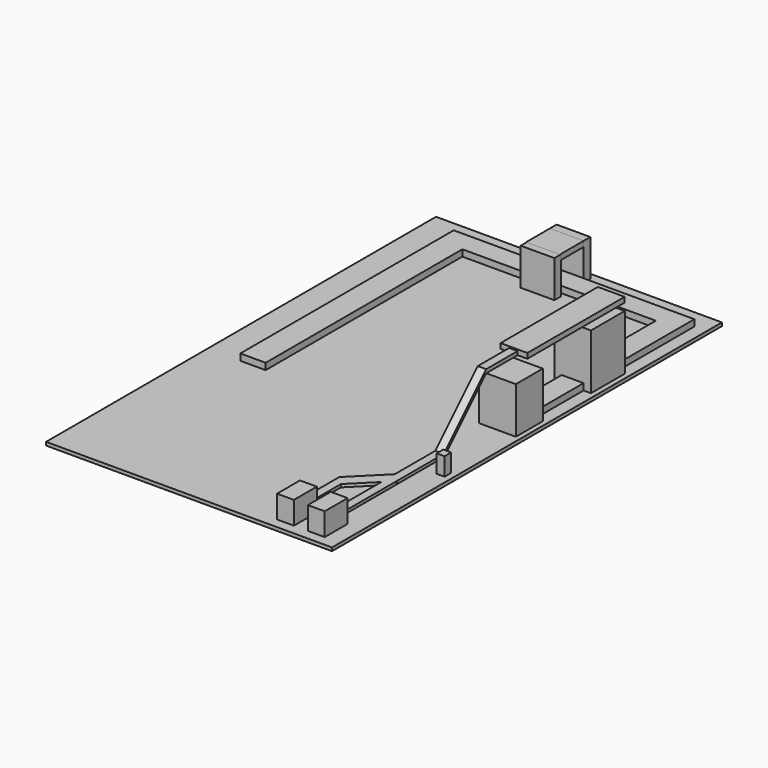
from build123d import *

# Parameters (mm, degrees)
F0_W         = 25.4
F0_H         = 43.18
F1_DEPTH     = 34.29
F4_DEPTH     = 186.69
F5_DEPTH     = 66.04
F6_SIZE      = 12.69999
F7_DEPTH     = 66.802
F8_W         = 11.9172371924
F8_H         = 12.5130861998
F9_DEPTH     = 27.178
F10_DEPTH    = 7.62
F11_T1_DEPTH = 38.8282991577
F12_W        = 12.7
F12_H        = 3.8690640952
F13_DEPTH    = 114.3
F14_T1_DEPTH = 38.8282991577
F15_DEPTH    = 59.182
F16_W        = 55.88
F16_H        = 50.8
F17_DEPTH    = 69.85
F19_DEPTH    = 91.186
F21_DEPTH    = 63.754
F22_DEPTH    = 208.788
F24_DEPTH    = 183.388
F25_DEPTH    = 179.07
F26_W        = 31.3697251636
F26_H        = 9.7994571552
F27_DEPTH    = 271.78
F28_DEPTH    = 58.166
F29_W        = 38.1454027963
F29_H        = 9.7994571552
F30_DEPTH    = 370.84
F31_W        = 50.8
F31_H        = 12.7
F32_DEPTH    = 55.88
F33_W        = 50.8
F33_H        = 8.1367950189
F34_DEPTH    = 44.704
F35_W        = 431.2671199441
F35_H        = 735.1557686925
F36_DEPTH    = 5.08


# Not quite as in the source:
# - a fillet or chamfer that OpenCascade refuses, or shapes differently, is made with other operations: its cross-section is extruded or revolved along the edge and cut away or added
# - a fillet or chamfer is up to 0.001 mm smaller than in the source, because OpenCascade refuses the exact size


with BuildPart() as f1:
    # F0 (on Top) → F1 (new body)
    with BuildSketch(Plane.XY):
        with Locations((-12.1586725817, -35.5092528684)):
            Rectangle(F0_W, F0_H)
    extrude(amount=F1_DEPTH)

    # F3 (on face) → F5 (join)
    with BuildSketch(Plane(origin=(0, -13.9192528684, 0), x_dir=(-1, 0, 0), z_dir=(0, 1, 0))):
        Polygon((12.1586725817, 13.97), (5.8086725817, 13.97), (5.8086725817, 9.525), (12.1586725817, 9.525), (18.5086725817, 9.525), (18.5086725817, 11.7475), (18.5086725817, 13.97), align=None)
    extrude(amount=F5_DEPTH)

    # F6 (size 12.7 in the source; OpenCascade refuses exactly that, so slightly less here)
    f6_edges = [f1.edges().sort_by_distance(p)[0] for p in [
        (-5.808673, 52.120747, 11.7475),
    ]]
    chamfer(f6_edges, length=F6_SIZE)

    # F7 (add): a face of the model
    f7_faces = [f1.faces().sort_by_distance(p)[0] for p in [
        (-12.1586675817, 45.7707521316, 11.7475),
    ]]


with BuildPart() as f1b:
    # F0 (on Top) → F1, piece 2 (new body)
    with BuildSketch(Plane.XY):
        with Locations((34.3718913153, -35.5737248565)):
            Rectangle(F0_W, F0_H)
    extrude(amount=F1_DEPTH)

    # F2 (on face) → F4 (join)
    with BuildSketch(Plane(origin=(0, -13.9837248565, 0), x_dir=(-1, 0, 0), z_dir=(0, 1, 0))):
        Polygon((-34.3718913153, 13.97), (-40.7218913153, 13.97), (-40.7218913153, 9.525), (-34.3718913153, 9.525), (-28.0218913153, 9.525), (-28.0218913153, 11.7475), (-28.0218913153, 13.97), align=None)
    extrude(amount=F4_DEPTH)


with BuildPart() as f1_1:
    add(f1.part)

    add(f1b.part)  # F7 merges F1b
    extrude(f7_faces, amount=F7_DEPTH)

    # F10 (add): a face of the model
    f10_faces = [f1_1.faces().sort_by_distance(p)[0] for p in [
        (34.3718913153, 172.7062751435, 11.7475),
    ]]
    extrude(f10_faces, amount=F10_DEPTH)

    # F11: chamfer of 5.08 on 1 edges, made by hand

    # F11_s2 → F11_t1 (cut)
    with BuildSketch(Plane.YZ.offset(14.9577417365)):
        Polygon((175.2462751435, 13.97), (180.3262751435, 8.89), (180.3262751435, 13.97), align=None)
    extrude(amount=F11_T1_DEPTH, mode=Mode.SUBTRACT)

    # F12 (on face) → F13 (join)
    with BuildSketch(Plane(origin=(0, 94.6081375717, 94.6081375717), x_dir=(1, 0, 0), z_dir=(0, 0.7071067812, 0.7071067812))):
        with Locations((34.3718913153, 115.9740798461)):
            Rectangle(F12_W, F12_H)
    extrude(amount=F13_DEPTH)

    # F14: chamfer of 5.08 on 1 edges, made by hand

    # F14_s2 → F14_t1 (cut)
    with BuildSketch(Plane.YZ.offset(14.9577417365)):
        Polygon((255.2123192432, 88.4643611826), (255.2123192432, 95.6485660795), (258.8044216917, 92.0564636311), align=None)
    extrude(amount=F14_T1_DEPTH, mode=Mode.SUBTRACT)

    # F15 (add): a face of the model
    f15_faces = [f1_1.faces().sort_by_distance(p)[0] for p in [
        (34.3718913153, 255.2123192432, 91.2002026412),
    ]]
    extrude(f15_faces, amount=F15_DEPTH)


with BuildPart() as f9:
    # F8 (on Top) → F9 (new body)
    with BuildSketch(Plane.XY):
        with Locations((55.1246125251, 157.5556769967)):
            Rectangle(F8_W, F8_H)
    extrude(amount=F9_DEPTH)


with BuildPart() as f17:
    # F16 (on Top) → F17 (new body)
    with BuildSketch(Plane.XY):
        with Locations((35.0235989317, 308.7478742687)):
            Rectangle(F16_W, F16_H)
    extrude(amount=F17_DEPTH)

    # F18 (on face) → F19 (join)
    with BuildSketch(Plane(origin=(0, 334.1478742687, 0), x_dir=(-1, 0, 0), z_dir=(0, 1, 0))):
        Polygon((-51.5335989317, 4.8997285776), (-51.5335989317, 0), (-18.5135989317, 0), (-18.5135989317, 4.8997285776), (-18.5135989317, 9.7994571552), (-51.5335989317, 9.7994571552), align=None)
    extrude(amount=F19_DEPTH)


with BuildPart() as f21:
    # F20 (on face) → F21 (new body)
    with BuildSketch(Plane(origin=(0, 425.3338742687, 0), x_dir=(-1, 0, 0), z_dir=(0, 1, 0))):
        Polygon((-7.8530972824, 83.3608135581), (-62.7023540437, 83.3608135581), (-62.7023540437, 0), (-51.5335989317, 0), (-51.5335989317, 9.7994571552), (-18.5135989317, 9.7994571552), (-18.5135989317, 0), (-7.8530972824, 0), align=None)
    extrude(amount=F21_DEPTH)


with BuildPart() as f22:
    # F22 (new): a face of the model
    f22_faces = [f17.part.faces().sort_by_distance(p)[0] for p in [
        (35.0235989317, 425.3338742687, 4.8997285776),
    ]]
    extrude(f22_faces, amount=F22_DEPTH)

    # F26 (on face) → F27 (join)
    with BuildSketch(Plane(origin=(18.5135989317, 0, 0), x_dir=(0, -1, 0), z_dir=(-1, 0, 0))):
        with Locations((-618.4370116869, 4.8997285776)):
            Rectangle(F26_W, F26_H)
    extrude(amount=F27_DEPTH)

    # F28 (add): a face of the model
    f28_faces = [f22.faces().sort_by_distance(p)[0] for p in [
        (-253.2664010683, 618.4370116869, 4.8997285776),
    ]]
    extrude(f28_faces, amount=F28_DEPTH)

    # F29 (on face) → F30 (join)
    with BuildSketch(Plane.XZ.offset(-602.7521491051)):
        with Locations((-292.3596996701, 4.8997285776)):
            Rectangle(F29_W, F29_H)
    extrude(amount=F30_DEPTH)


with BuildPart() as f24:
    # F23 (on face) → F24 (new body)
    with BuildSketch(Plane(origin=(0, 314.3943192432, 0), x_dir=(-1, 0, 0), z_dir=(0, 1, 0))):
        Polygon((-15.1371452957, 96.2249219918), (-55.5143468082, 96.2249219918), (-55.5143468082, 88.4643611826), (-40.7218913153, 88.4643611826), (-40.7218913153, 93.9360440997), (-28.0218913153, 93.9360440997), (-28.0218913153, 88.4643611826), (-15.1371452957, 88.4643611826), align=None)
    extrude(amount=F24_DEPTH)


with BuildPart() as f25:
    # F25 (new): a face of the model
    f25_faces = [f1_1.part.faces().sort_by_distance(p)[0] for p in [
        (34.3718913153, 314.3943192432, 91.2002026412),
    ]]
    extrude(f25_faces, amount=F25_DEPTH)


with BuildPart() as f32:
    # F31 (on Top) → F32 (new body)
    with BuildSketch(Plane.XY):
        with Locations((-145.2229168913, 645.8647573679)):
            Rectangle(F31_W, F31_H)
    extrude(amount=F32_DEPTH)


with BuildPart() as f32b:
    # F31 (on Top) → F32, piece 2 (new body)
    with BuildSketch(Plane.XY):
        with Locations((-144.5784862739, 590.0489869958)):
            Rectangle(F31_W, F31_H)
    extrude(amount=F32_DEPTH)


with BuildPart() as f34:
    # F33 (on face) → F34 (new body)
    with BuildSketch(Plane.XZ.offset(-639.5147573679)):
        with Locations((-145.2229168913, 51.8116024905)):
            Rectangle(F33_W, F33_H)
    extrude(amount=F34_DEPTH)


with BuildPart() as f36:
    # F35 (on Top) → F36 (new body)
    with BuildSketch(Plane.XY):
        with Locations((-145.4154662788, 295.2351234853)):
            Rectangle(F35_W, F35_H)
    extrude(amount=-F36_DEPTH)


solid = Compound([f1_1.part, f9.part, f17.part, f21.part, f22.part, f24.part, f25.part, f32.part, f32b.part, f34.part, f36.part])
